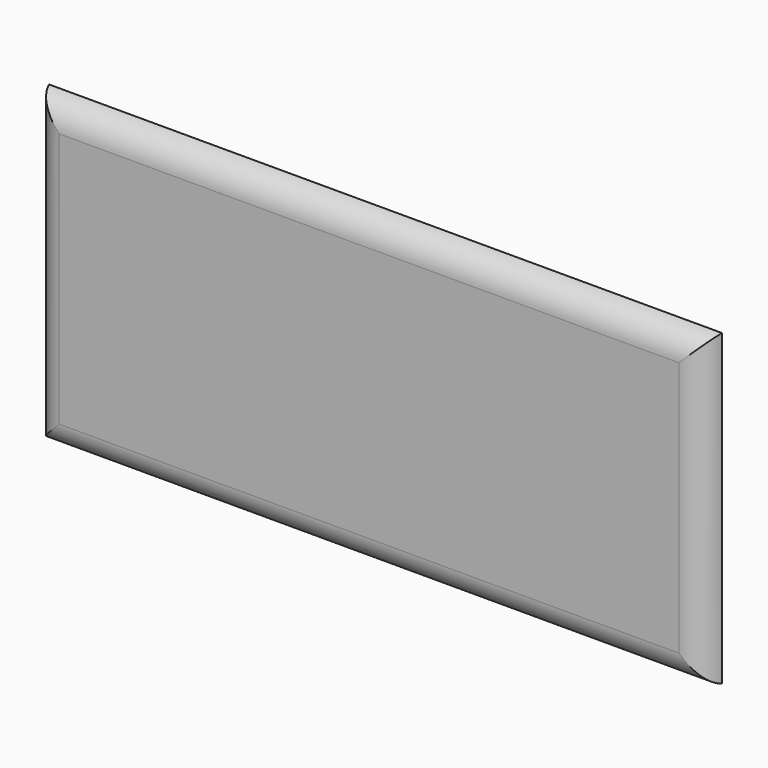
from build123d import *

# Parameters (mm, degrees)
F0_W        = 124.8843446374
F0_H        = 57.2863984853
F1_DEPTH    = 3.81
F2_T1_DEPTH = 149.4777888858
F2_T3_DEPTH = 81.8798427337


# Not quite as in the source:
# - a fillet or chamfer that OpenCascade refuses, or shapes differently, is made with other operations: its cross-section is extruded or revolved along the edge and cut away or added


with BuildPart() as f1:
    # F0 (on Front) → F1 (new body)
    with BuildSketch(Plane.XZ):
        with Locations((2.9597990215, -0.095478259)):
            Rectangle(F0_W, F0_H)
    extrude(amount=F1_DEPTH)

    # F2: fillet of radius 5.08 on 4 edges, made by hand

    # F2_s2 → F2_t1 (cut)
    with BuildSketch(Plane.YZ.offset(-71.7790954214)):
        with BuildLine():
            ThreePointArc((0, 28.5477209836), (-2.7460926284, 26.7398841073), (-3.81, 23.6290321339))
            Line((-3.81, 23.6290321339), (-3.81, 28.5477209836))
            Line((-3.81, 28.5477209836), (0, 28.5477209836))
        make_face()
        with BuildLine():
            ThreePointArc((0, -28.7386775017), (-2.7460926284, -26.9308406253), (-3.81, -23.819988652))
            Line((-3.81, -23.819988652), (-3.81, -28.7386775017))
            Line((-3.81, -28.7386775017), (0, -28.7386775017))
        make_face()
    extrude(amount=F2_T1_DEPTH, mode=Mode.SUBTRACT)

    # F2_s4 → F2_t3 (cut)
    with BuildSketch(Plane.XY.offset(-41.0353996259)):
        with BuildLine():
            ThreePointArc((-59.4823732972, 0), (-57.6745364209, -2.7460926284), (-54.5636844475, -3.81))
            Line((-54.5636844475, -3.81), (-59.4823732972, -3.81))
            Line((-59.4823732972, -3.81), (-59.4823732972, 0))
        make_face()
        with BuildLine():
            ThreePointArc((65.4019713402, 0), (63.5941344638, -2.7460926284), (60.4832824905, -3.81))
            Line((60.4832824905, -3.81), (65.4019713402, -3.81))
            Line((65.4019713402, -3.81), (65.4019713402, 0))
        make_face()
    extrude(amount=F2_T3_DEPTH, mode=Mode.SUBTRACT)


solid = f1.part
